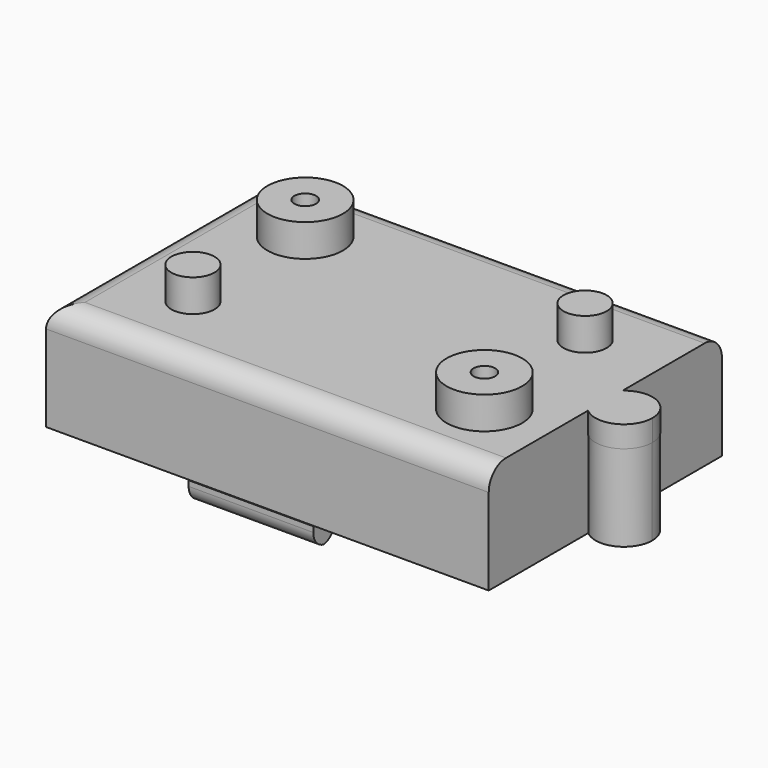
from build123d import *

# Parameters (mm, degrees)
F0_W         = 37
F0_H         = 23
F0_R         = 1.4922705886
F1_DEPTH     = 8
F3_D         = 3
F3_DEPTH     = 4
F3_TIP       = 0.9012909285
F5_DEPTH     = 2
F6_R         = 2
F7_W         = 11.5434788167
F7_H         = 2.4902373552
F8_DEPTH     = 2
F9_T1_DEPTH  = 19.0434788167
F10_T1_DEPTH = 19.0434788167
F11_R        = 3.5
F11_R_2      = 1
F11_R_3      = 2
F12_DEPTH    = 3


# Not quite as in the source:
# - a fillet or chamfer that OpenCascade refuses, or shapes differently, is made with other operations: its cross-section is extruded or revolved along the edge and cut away or added


with BuildPart() as f1:
    # F0 (on Top) → F1 (new body)
    with BuildSketch(Plane.XY):
        with BuildLine():
            Line((-10.4036603272, 27), (-51.4036603272, 27))
            Line((-51.4036603272, 27), (-51.4036603272, 0))
            Line((-51.4036603272, 0), (-10.4036603272, 0))
            Line((-10.4036603272, 0), (-10.4036603272, 11.5282175104))
            ThreePointArc((-10.4036603272, 11.5282175104), (-11.2988558778, 13.5), (-10.4036603272, 15.4717824896))
            Line((-10.4036603272, 15.4717824896), (-10.4036603272, 27))
        make_face()
        with Locations((-30.9036603272, 13.5)):
            Rectangle(F0_W, F0_H, mode=Mode.SUBTRACT)
        with BuildLine():
            ThreePointArc((-6.0605576566, 13.5), (-7.5969670408, 15.8848724805), (-10.4036603272, 15.4717824896))
            Line((-10.4036603272, 15.4717824896), (-10.4036603272, 11.5282175104))
            ThreePointArc((-10.4036603272, 11.5282175104), (-7.5969670408, 11.1151275195), (-6.0605576566, 13.5))
        make_face()
        with Locations((-8.6797067672, 13.5)):
            Circle(F0_R, mode=Mode.SUBTRACT)
        with BuildLine():
            Line((-10.4036603272, 11.5282175104), (-10.4036603272, 15.4717824896))
            ThreePointArc((-10.4036603272, 15.4717824896), (-11.2988558778, 13.5), (-10.4036603272, 11.5282175104))
        make_face()
    extrude(amount=F1_DEPTH)

    # F3 (one way)
    with BuildSketch(Plane(origin=(-12.4036603272, 0, 0), x_dir=(0, -1, 0), z_dir=(-1, 0, 0))):
        with Locations((-13.5, 4)):
            Circle(F3_D / 2)
    extrude(amount=-F3_DEPTH, mode=Mode.SUBTRACT)
    with Locations(Plane(origin=(-12.4036603272, 0, 0), x_dir=(0, -1, 0), z_dir=(-1, 0, 0))):
        with Locations((-13.5, 4)):
            with Locations((0, 0, -(F3_DEPTH + F3_TIP / 2))):  # 118° drill point
                Cone(0, F3_D / 2, F3_TIP, mode=Mode.SUBTRACT)

    # F4 (on face) → F5 (join)
    with BuildSketch(Plane.XY.offset(8)):
        with BuildLine():
            Line((-10.4036603272, 27), (-51.4036603272, 27))
            Line((-51.4036603272, 27), (-51.4036603272, 0))
            Line((-51.4036603272, 0), (-10.4036603272, 0))
            Line((-10.4036603272, 0), (-10.4036603272, 11.4980807802))
            ThreePointArc((-10.4036603272, 11.4980807802), (-11.3216182797, 13.5), (-10.4036603272, 15.5019192198))
            Line((-10.4036603272, 15.5019192198), (-10.4036603272, 27))
        make_face()
        with BuildLine():
            ThreePointArc((-6.0377952547, 13.5), (-7.5785338283, 15.9014817506), (-10.4036603272, 15.5019192198))
            Line((-10.4036603272, 15.5019192198), (-10.4036603272, 11.4980807802))
            ThreePointArc((-10.4036603272, 11.4980807802), (-7.5785338283, 11.0985182494), (-6.0377952547, 13.5))
        make_face()
        with BuildLine():
            Line((-10.4036603272, 11.4980807802), (-10.4036603272, 15.5019192198))
            ThreePointArc((-10.4036603272, 15.5019192198), (-11.3216182797, 13.5), (-10.4036603272, 11.4980807802))
        make_face()
    extrude(amount=F5_DEPTH)

    # F6
    f6_edges = [f1.edges().sort_by_distance(p)[0] for p in [
        (-51.40366, 13.5, 10),
        (-30.90366, 27, 10),
        (-30.90366, 0, 10),
    ]]
    fillet(f6_edges, radius=F6_R)

    # F7 (on Top) → F8 (join)
    with BuildSketch(Plane.XY):
        with Locations((-32.3717817664, 1.1760484776)):
            Rectangle(F7_W, F7_H)
        with Locations((-32.1847852319, 25.1162685454)):
            Rectangle(F7_W, F7_H)
    extrude(amount=-F8_DEPTH)

    # F9: fillet of radius 1.5 on 2 edges, made by hand

    # F9_s2 → F9_t1 (cut)
    with BuildSketch(Plane.YZ.offset(-41.7065246403)):
        with BuildLine():
            ThreePointArc((26.361387223, -0.5), (25.9220473948, -1.5606601718), (24.861387223, -2))
            Line((24.861387223, -2), (26.361387223, -2))
            Line((26.361387223, -2), (26.361387223, -0.5))
        make_face()
        with BuildLine():
            ThreePointArc((23.8711498678, -0.5), (24.310489696, -1.5606601718), (25.3711498678, -2))
            Line((25.3711498678, -2), (23.8711498678, -2))
            Line((23.8711498678, -2), (23.8711498678, -0.5))
        make_face()
    extrude(amount=F9_T1_DEPTH, mode=Mode.SUBTRACT)

    # F10: fillet of radius 1.5 on 2 edges, made by hand

    # F10_s2 → F10_t1 (cut)
    with BuildSketch(Plane.YZ.offset(-41.8935211748)):
        with BuildLine():
            ThreePointArc((2.4211671553, -0.5), (1.981827327, -1.5606601718), (0.9211671553, -2))
            Line((0.9211671553, -2), (2.4211671553, -2))
            Line((2.4211671553, -2), (2.4211671553, -0.5))
        make_face()
        with BuildLine():
            ThreePointArc((-0.0690702, -0.5), (0.3702696283, -1.5606601718), (1.4309298, -2))
            Line((1.4309298, -2), (-0.0690702, -2))
            Line((-0.0690702, -2), (-0.0690702, -0.5))
        make_face()
    extrude(amount=F10_T1_DEPTH, mode=Mode.SUBTRACT)

    # F11 (on face) → F12 (join)
    with BuildSketch(Plane.XY.offset(10)):
        with Locations((-16.4036603272, 7)):
            Circle(F11_R)
        with Locations((-16.4036603272, 7)):
            Circle(F11_R_2, mode=Mode.SUBTRACT)
        with Locations((-43.4036603272, 7)):
            Circle(F11_R_3)
        with Locations((-43.4036603272, 20)):
            Circle(F11_R)
        with Locations((-43.4036603272, 20)):
            Circle(F11_R_2, mode=Mode.SUBTRACT)
        with Locations((-17.4769777805, 20)):
            Circle(F11_R_3)
    extrude(amount=F12_DEPTH)


solid = f1.part
